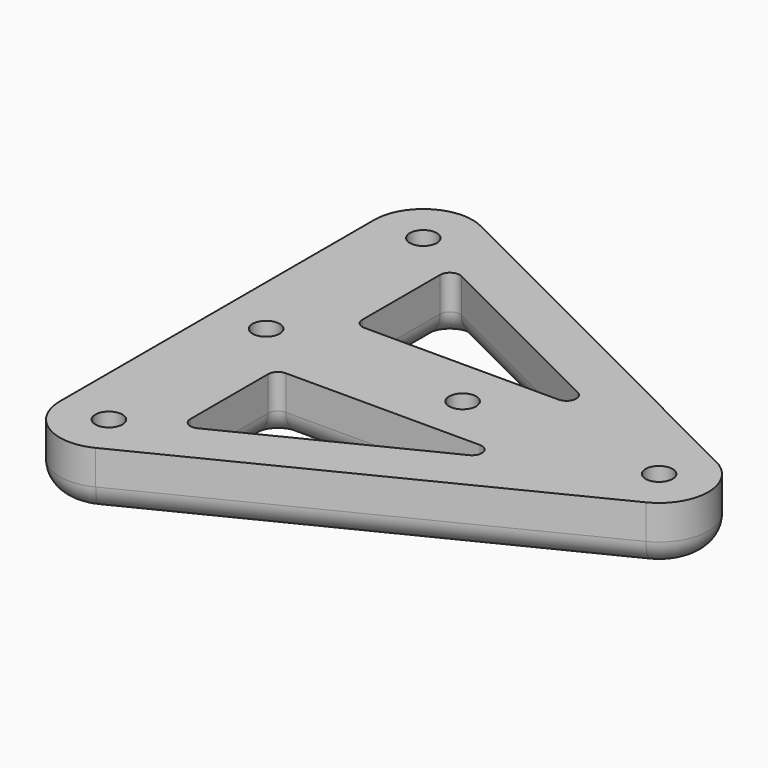
from build123d import *

# Parameters (mm, degrees)
F1_DEPTH       = 12
F2_D           = 5.5
F2_CBORE_D     = 9.75
F2_CBORE_DEPTH = 5
F3_R           = 4.99999


# Not quite as in the source:
# - a fillet or chamfer is up to 0.001 mm smaller than in the source, because OpenCascade refuses the exact size


with BuildPart() as f1:
    # F0 (on Top) → F1 (new body)
    with BuildSketch(Plane.XY):
        with BuildLine():
            Line((84.472135955, 8.94427191), (4.472135955, 48.94427191))
            ThreePointArc((4.472135955, 48.94427191), (-5.2573111212, 48.5065080835), (-10, 40))
            Line((-10, 40), (-10, -40))
            ThreePointArc((-10, -40), (-5.2573111212, -48.5065080835), (4.472135955, -48.94427191))
            Line((4.472135955, -48.94427191), (84.472135955, -8.94427191))
            ThreePointArc((84.472135955, -8.94427191), (90, 0), (84.472135955, 8.94427191))
        make_face()
        with BuildLine():
            Line((10, -31.7639320225), (10, -12))
            ThreePointArc((10, -12), (10.5857864376, -10.5857864376), (12, -10))
            Line((12, -10), (51.527864045, -10))
            ThreePointArc((51.527864045, -10), (53.4743620239, -11.5404941589), (52.422291236, -13.788854382))
            Line((52.422291236, -13.788854382), (12.894427191, -33.5527864045))
            ThreePointArc((12.894427191, -33.5527864045), (10.9485377758, -33.4652336392), (10, -31.7639320225))
        make_face(mode=Mode.SUBTRACT)
        with BuildLine():
            ThreePointArc((10, 31.7639320225), (10.9485377758, 33.4652336392), (12.894427191, 33.5527864045))
            Line((12.894427191, 33.5527864045), (52.422291236, 13.788854382))
            ThreePointArc((52.422291236, 13.788854382), (53.4743620239, 11.5404941589), (51.527864045, 10))
            Line((51.527864045, 10), (12, 10))
            ThreePointArc((12, 10), (10.5857864376, 10.5857864376), (10, 12))
            Line((10, 12), (10, 31.7639320225))
        make_face(mode=Mode.SUBTRACT)
    extrude(amount=F1_DEPTH)

    # F2 (through all)
    with Locations(Plane(origin=(0, 0, 0), x_dir=(1, 0, 0), z_dir=(0, 0, -1))):
        with Locations((0, -40), (0, 40), (0, 0), (40, 0), (80, 0)):
            CounterBoreHole(F2_D / 2, F2_CBORE_D / 2, F2_CBORE_DEPTH)

    # F3 (radius 5 in the source; OpenCascade refuses exactly that, so slightly less here)
    f3_edges = [f1.edges().sort_by_distance(p)[0] for p in [
        (44.472136, 28.944272, 0),
        (32.658359, 23.67082, 0),
        (32.658359, -23.67082, 0),
    ]]
    fillet(f3_edges, radius=F3_R)


solid = f1.part
